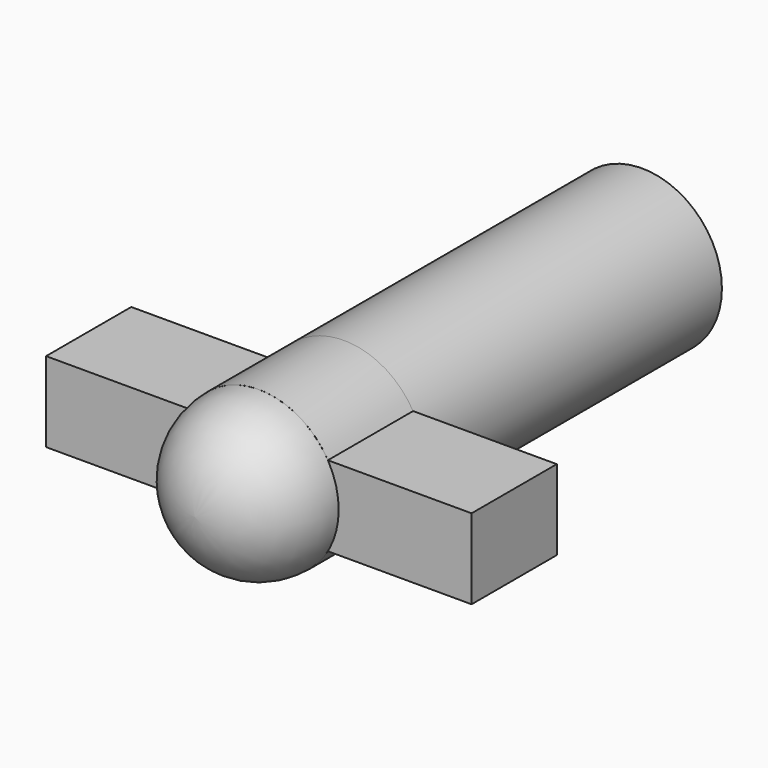
from build123d import *

# Parameters (mm, degrees)
F0_R     = 1.5
F1_DEPTH = 7
F3_DEPTH = 2
F4_R     = 1.5
F5_DEPTH = 1.5
F6_R     = 1.49999


# Not quite as in the source:
# - a fillet or chamfer is up to 0.001 mm smaller than in the source, because OpenCascade refuses the exact size


with BuildPart() as f1:
    # F0 (on Front) → F1 (new body)
    with BuildSketch(Plane.XZ):
        Circle(F0_R)
    extrude(amount=F1_DEPTH)

    # F2 (on face) → F3 (join)
    with BuildSketch(Plane.XZ.offset(7)):
        with BuildLine():
            ThreePointArc((1.2976046011, -0.752477441), (1.4485176736, -0.3896107662), (1.5, 0))
            ThreePointArc((1.5, 0), (1.4485176736, 0.3896107662), (1.2976046011, 0.752477441))
            Line((1.2976046011, 0.752477441), (-1.2976046011, 0.752477441))
            ThreePointArc((-1.2976046011, 0.752477441), (-1.5, 0), (-1.2976046011, -0.752477441))
            Line((-1.2976046011, -0.752477441), (1.2976046011, -0.752477441))
        make_face()
        with BuildLine():
            ThreePointArc((1.2976046011, 0.752477441), (1.4485176736, 0.3896107662), (1.5, 0))
            ThreePointArc((1.5, 0), (1.4485176736, -0.3896107662), (1.2976046011, -0.752477441))
            Line((1.2976046011, -0.752477441), (3.9969966747, -0.752477441))
            Line((3.9969966747, -0.752477441), (3.9969966747, 0.752477441))
            Line((3.9969966747, 0.752477441), (1.2976046011, 0.752477441))
        make_face()
        with BuildLine():
            Line((-1.2976046011, 0.752477441), (1.2976046011, 0.752477441))
            ThreePointArc((1.2976046011, 0.752477441), (0, 1.5), (-1.2976046011, 0.752477441))
        make_face()
        with BuildLine():
            ThreePointArc((-1.2976046011, -0.752477441), (0, -1.5), (1.2976046011, -0.752477441))
            Line((1.2976046011, -0.752477441), (-1.2976046011, -0.752477441))
        make_face()
        with BuildLine():
            ThreePointArc((-1.2976046011, -0.752477441), (-1.5, 0), (-1.2976046011, 0.752477441))
            Line((-1.2976046011, 0.752477441), (-3.9969966747, 0.752477441))
            Line((-3.9969966747, 0.752477441), (-3.9969966747, -0.752477441))
            Line((-3.9969966747, -0.752477441), (-1.2976046011, -0.752477441))
        make_face()
    extrude(amount=F3_DEPTH)

    # F4 (on face) → F5 (join)
    with BuildSketch(Plane.XZ.offset(9)):
        Circle(F4_R)
    extrude(amount=F5_DEPTH)

    # F6 (radius 1.5 in the source; OpenCascade refuses exactly that, so slightly less here)
    f6_edges = [f1.edges().sort_by_distance(p)[0] for p in [
        (-1.5, -10.5, 0),
    ]]
    fillet(f6_edges, radius=F6_R)


solid = f1.part
